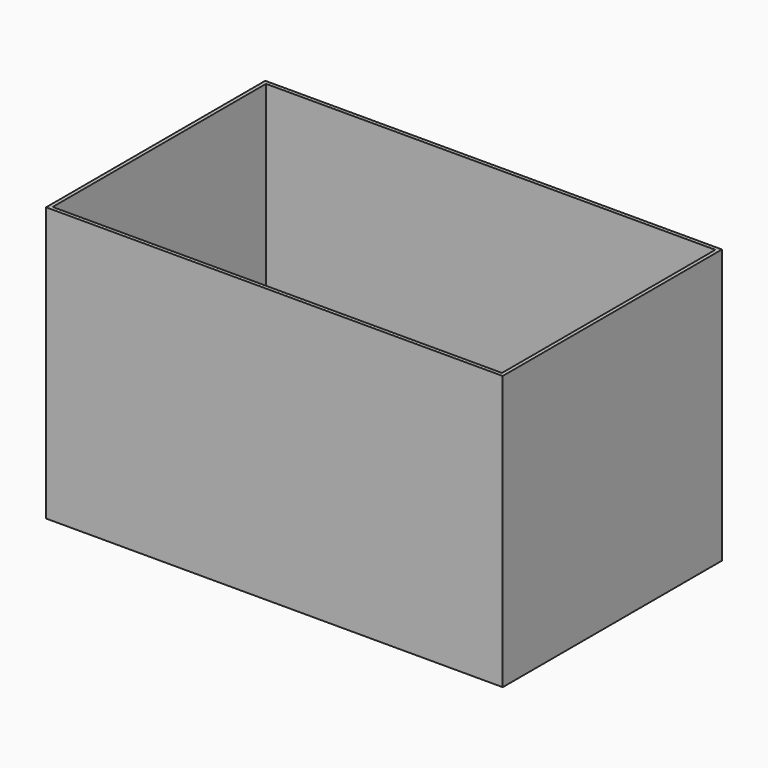
from build123d import *

# Parameters (mm, degrees)
F1_W     = 246
F1_H     = 146
F1_W_2   = 10
F1_H_2   = 130
F2_DEPTH = 6
F3_DEPTH = 150


# Not quite as in the source:
# - ends of sketch curves that miss each other by under 0.0002 mm in the source are joined


with BuildPart() as f2:
    # F1 (on face) → F2 (new body)
    with BuildSketch(Plane.XY):
        with Locations((-18.3215842792, -1.6598337144)):
            Rectangle(F1_W, F1_H)
        with Locations((-128.3215842792, -1.6598337144)):
            Rectangle(F1_W_2, F1_H_2, mode=Mode.SUBTRACT)
        with Locations((-108.3215842792, -1.6598337144)):
            Rectangle(F1_W_2, F1_H_2, mode=Mode.SUBTRACT)
        with Locations((-88.3215842792, -1.6598337144)):
            Rectangle(F1_W_2, F1_H_2, mode=Mode.SUBTRACT)
        with Locations((-68.3215842792, -1.6598337144)):
            Rectangle(F1_W_2, F1_H_2, mode=Mode.SUBTRACT)
        with Locations((-48.3215842792, -1.6598337144)):
            Rectangle(F1_W_2, F1_H_2, mode=Mode.SUBTRACT)
        with Locations((-28.3215842792, -1.6598337144)):
            Rectangle(F1_W_2, F1_H_2, mode=Mode.SUBTRACT)
        with Locations((-8.3215842792, -1.6598337144)):
            Rectangle(F1_W_2, F1_H_2, mode=Mode.SUBTRACT)
        with Locations((11.6784157208, -1.6598337144)):
            Rectangle(F1_W_2, F1_H_2, mode=Mode.SUBTRACT)
        with Locations((31.6784157208, -1.6598337144)):
            Rectangle(F1_W_2, F1_H_2, mode=Mode.SUBTRACT)
        with Locations((51.6784157208, -1.6598337144)):
            Rectangle(F1_W_2, F1_H_2, mode=Mode.SUBTRACT)
        with Locations((71.6784157208, -1.6598337144)):
            Rectangle(F1_W_2, F1_H_2, mode=Mode.SUBTRACT)
        with Locations((91.6784157208, -1.6598337144)):
            Rectangle(F1_W_2, F1_H_2, mode=Mode.SUBTRACT)
    extrude(amount=F2_DEPTH)

    # F1 (on face) → F3 (join)
    with BuildSketch(Plane.XY):
        Polygon((106.6783964634, -76.6597911716), (106.6783964634, 73.3401662856), (-143.3215842792, 73.3401662856), (-143.3215842792, -76.6598337144), align=None)
        with Locations((-18.3215842792, -1.6598337144)):
            Rectangle(F1_W, F1_H, mode=Mode.SUBTRACT)
    extrude(amount=F3_DEPTH)


solid = f2.part
